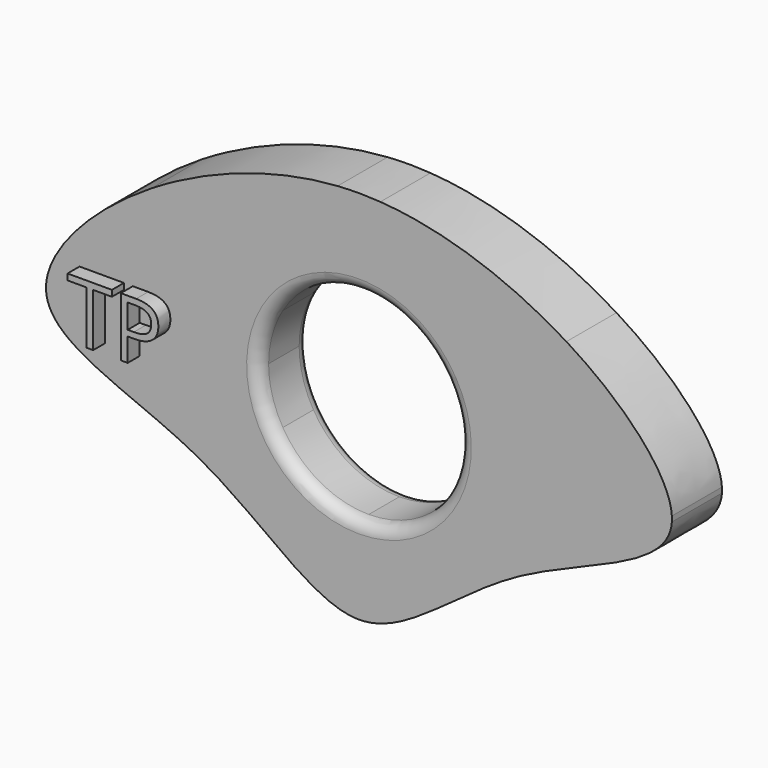
from build123d import *

# Parameters (mm, degrees)
F1_DEPTH     = 6.35
F3_TEXT_SIZE = 8.4123936378
F4_DEPTH     = 7.874


# Not quite as in the source:
# - a fillet or chamfer that OpenCascade refuses, or shapes differently, is made with other operations: its cross-section is extruded or revolved along the edge and cut away or added
# - Text() gives the source's letters only with a copy of the font that has no kerning and outlines rounded to 1/6400 em; it was checked with that copy


with BuildPart() as f1:
    # F0 (on Front) → F1 (new body)
    with BuildSketch(Plane.XZ):
        with BuildLine():
            add(Edge.make_bspline(
                [(-31.75, -38.1), (-26.9196709524, -38.1), (-22.0893419047, -32.5027306314), (-15.3722677145, -28.8766393713)],
                knots=[0.2929135327, 0.2929135327, 0.2929135327, 0.2929135327, 0.4404608065, 0.4404608065, 0.4404608065, 0.4404608065], degree=3))
            Line((-15.3722677145, -28.8766393713), (-23.0378718748, -24.2772768751))
            ThreePointArc((-23.0378718748, -24.2772768751), (-26.7441800398, -27.8912310526), (-31.75, -29.21))
            Line((-31.75, -29.21), (-31.75, -38.1))
        make_face()
        with BuildLine():
            ThreePointArc((-15.3722677145, -28.8766393713), (-13.3434748609, -24.148312314), (-12.6504461794, -19.05))
            Line((-12.6504461794, -19.05), (-21.59, -19.05))
            ThreePointArc((-21.59, -19.05), (-21.9586563294, -21.7620451921), (-23.0378718748, -24.2772768751))
            Line((-23.0378718748, -24.2772768751), (-15.3722677145, -28.8766393713))
        make_face()
        with BuildLine():
            add(Edge.make_bspline(
                [(-15.3722677145, -28.8766393713), (-8.7544839905, -25.3041482772), (-0.3053218561, -23.6449908652), (0, -19.05)],
                knots=[0.4404608065, 0.4404608065, 0.4404608065, 0.4404608065, 0.5858270655, 0.5858270655, 0.5858270655, 0.5858270655], degree=3))
            Line((0, -19.05), (-12.6504461794, -19.05))
            ThreePointArc((-12.6504461794, -19.05), (-13.3434748609, -24.148312314), (-15.3722677145, -28.8766393713))
        make_face()
        with BuildLine():
            Line((0, -19.05), (0, -18.5163144511))
            add(Edge.make_bspline(
                [(0, -18.5163144511), (-0.2161143448, -15.0824614861), (-4.4759800562, -10.2742950568), (-10.6970013922, -6.4182008353)],
                knots=[0.5913256791, 0.5913256791, 0.5913256791, 0.5913256791, 0.6951466037, 0.6951466037, 0.6951466037, 0.6951466037], degree=3))
            Line((-10.6970013922, -6.4182008353), (-15.3722677145, -9.2233606287))
            ThreePointArc((-15.3722677145, -9.2233606287), (-13.3434748609, -13.951687686), (-12.6504461794, -19.05))
            Line((-12.6504461794, -19.05), (0, -19.05))
        make_face()
        with BuildLine():
            ThreePointArc((-12.6504461794, -19.05), (-13.3434748609, -13.951687686), (-15.3722677145, -9.2233606287))
            Line((-15.3722677145, -9.2233606287), (-23.0378718748, -13.8227231249))
            ThreePointArc((-23.0378718748, -13.8227231249), (-21.9586563294, -16.3379548079), (-21.59, -19.05))
            Line((-21.59, -19.05), (-12.6504461794, -19.05))
        make_face()
        with BuildLine():
            add(Edge.make_bspline(
                [(-29.5779776849, -0.0743504667), (-30.3009796307, -0.025345087), (-31.0254898153, 0), (-31.75, 0)],
                knots=[0.783590155, 0.783590155, 0.783590155, 0.783590155, 0.7929135327, 0.7929135327, 0.7929135327, 0.7929135327], degree=3))
            Line((-31.75, 0), (-31.75, -8.89))
            ThreePointArc((-31.75, -8.89), (-26.7441800398, -10.2087689474), (-23.0378718748, -13.8227231249))
            Line((-23.0378718748, -13.8227231249), (-15.3722677145, -9.2233606287))
            ThreePointArc((-15.3722677145, -9.2233606287), (-21.4083634916, -2.9924936408), (-29.5779776849, -0.0743504667))
        make_face()
        with BuildLine():
            Line((-31.75, -8.89), (-31.75, 0))
            add(Edge.make_bspline(
                [(-31.75, 0), (-32.4745101847, 0), (-33.1990203693, -0.025345087), (-33.9220223151, -0.0743504667)],
                knots=[0.7929135327, 0.7929135327, 0.7929135327, 0.7929135327, 0.8022369105, 0.8022369105, 0.8022369105, 0.8022369105], degree=3))
            ThreePointArc((-33.9220223151, -0.0743504667), (-42.0916365084, -2.9924936408), (-48.1277322855, -9.2233606287))
            Line((-48.1277322855, -9.2233606287), (-40.4621281252, -13.8227231249))
            ThreePointArc((-40.4621281252, -13.8227231249), (-36.7558199602, -10.2087689474), (-31.75, -8.89))
        make_face()
        with BuildLine():
            ThreePointArc((-50.8495538206, -19.05), (-50.1565251391, -13.951687686), (-48.1277322855, -9.2233606287))
            Line((-48.1277322855, -9.2233606287), (-52.8029986078, -6.4182008353))
            add(Edge.make_bspline(
                [(-52.8029986078, -6.4182008353), (-59.0240199438, -10.2742950568), (-63.2838856552, -15.0824614861), (-63.5, -18.5163144511)],
                knots=[0.8906804618, 0.8906804618, 0.8906804618, 0.8906804618, 0.9945013864, 0.9945013864, 0.9945013864, 0.9945013864], degree=3))
            Line((-63.5, -18.5163144511), (-63.5, -19.05))
            Line((-63.5, -19.05), (-50.8495538206, -19.05))
        make_face()
        with BuildLine():
            ThreePointArc((-48.1277322855, -28.8766393713), (-50.1565251391, -24.148312314), (-50.8495538206, -19.05))
            Line((-50.8495538206, -19.05), (-63.5, -19.05))
            add(Edge.make_bspline(
                [(-63.5, -19.05), (-63.1946781439, -23.6449908652), (-54.7455160095, -25.3041482772), (-48.1277322855, -28.8766393713)],
                knots=[0, 0, 0, 0, 0.145366259, 0.145366259, 0.145366259, 0.145366259], degree=3))
        make_face()
        with BuildLine():
            Line((-48.1277322855, -28.8766393713), (-40.4621281252, -24.2772768751))
            ThreePointArc((-40.4621281252, -24.2772768751), (-41.5413436706, -21.7620451921), (-41.91, -19.05))
            Line((-41.91, -19.05), (-50.8495538206, -19.05))
            ThreePointArc((-50.8495538206, -19.05), (-50.1565251391, -24.148312314), (-48.1277322855, -28.8766393713))
        make_face()
        with BuildLine():
            ThreePointArc((-41.91, -19.05), (-41.5413436706, -16.3379548079), (-40.4621281252, -13.8227231249))
            Line((-40.4621281252, -13.8227231249), (-48.1277322855, -9.2233606287))
            ThreePointArc((-48.1277322855, -9.2233606287), (-50.1565251391, -13.951687686), (-50.8495538206, -19.05))
            Line((-50.8495538206, -19.05), (-41.91, -19.05))
        make_face()
        with BuildLine():
            add(Edge.make_bspline(
                [(-48.1277322855, -28.8766393713), (-41.4106580953, -32.5027306314), (-36.5803290476, -38.1), (-31.75, -38.1)],
                knots=[0.145366259, 0.145366259, 0.145366259, 0.145366259, 0.2929135327, 0.2929135327, 0.2929135327, 0.2929135327], degree=3))
            Line((-31.75, -38.1), (-31.75, -29.21))
            ThreePointArc((-31.75, -29.21), (-36.7558199602, -27.8912310526), (-40.4621281252, -24.2772768751))
            Line((-40.4621281252, -24.2772768751), (-48.1277322855, -28.8766393713))
        make_face()
        with BuildLine():
            Line((-15.3722677145, -9.2233606287), (-10.6970013922, -6.4182008353))
            add(Edge.make_bspline(
                [(-10.6970013922, -6.4182008353), (-15.9965999269, -3.1332496702), (-22.7194269191, -0.5392259577), (-29.5779776849, -0.0743504667)],
                knots=[0.6951466037, 0.6951466037, 0.6951466037, 0.6951466037, 0.783590155, 0.783590155, 0.783590155, 0.783590155], degree=3))
            ThreePointArc((-29.5779776849, -0.0743504667), (-21.4083634916, -2.9924936408), (-15.3722677145, -9.2233606287))
        make_face()
        with BuildLine():
            ThreePointArc((-48.1277322855, -9.2233606287), (-42.0916365084, -2.9924936408), (-33.9220223151, -0.0743504667))
            add(Edge.make_bspline(
                [(-33.9220223151, -0.0743504667), (-40.7805730809, -0.5392259577), (-47.5034000731, -3.1332496702), (-52.8029986078, -6.4182008353)],
                knots=[0.8022369105, 0.8022369105, 0.8022369105, 0.8022369105, 0.8906804618, 0.8906804618, 0.8906804618, 0.8906804618], degree=3))
            Line((-52.8029986078, -6.4182008353), (-48.1277322855, -9.2233606287))
        make_face()
    extrude(amount=F1_DEPTH)

    # F2: fillet of radius 1.27 on 2 edges, made by hand

    # F2_s1 → F2_t2 (revolve, cut)
    with BuildSketch(Plane.YZ.offset(-31.75)):
        with BuildLine():
            ThreePointArc((-5.0790343146, -29.2096), (-5.9780256121, -29.5819743879), (-6.3504, -30.4809656854))
            Line((-6.3504, -30.4809656854), (-6.4775365685, -30.4809656854))
            ThreePointArc((-6.4775365685, -30.4809656854), (-6.4771365685, -29.8454828427), (-6.4771365685, -29.21))
            Line((-6.4771365685, -29.21), (-6.35, -29.0828634315))
            ThreePointArc((-6.35, -29.0828634315), (-5.7145171573, -29.0828634315), (-5.0790343146, -29.0824634315))
            Line((-5.0790343146, -29.0824634315), (-5.0790343146, -29.2096))
        make_face()
    revolve(axis=Axis((-31.75, -6.35, -19.05), (0, 1, 0)), mode=Mode.SUBTRACT)

    # F2_s3 → F2_t4 (revolve, cut)
    with BuildSketch(Plane.YZ.offset(-31.75)):
        with BuildLine():
            ThreePointArc((-1.2709656854, -29.2096), (-0.3719743879, -29.5819743879), (0.0004, -30.4809656854))
            Line((0.0004, -30.4809656854), (0.1275365685, -30.4809656854))
            ThreePointArc((0.1275365685, -30.4809656854), (0.1271365685, -29.8454828427), (0.1271365685, -29.21))
            Line((0.1271365685, -29.21), (0, -29.0828634315))
            ThreePointArc((0, -29.0828634315), (-0.6354828427, -29.0828634315), (-1.2709656854, -29.0824634315))
            Line((-1.2709656854, -29.0824634315), (-1.2709656854, -29.2096))
        make_face()
    revolve(axis=Axis((-31.75, 0, -19.05), (0, 1, 0)), mode=Mode.SUBTRACT)

    # F3 (on Front) → F4 (join)
    with BuildSketch(Plane.XZ):
        with Locations((-60.1784624159, -21.7853859067)):
            Text('TP', F3_TEXT_SIZE, font='Open Sans', text_align=(TextAlign.LEFT, TextAlign.BOTTOM))
    extrude(amount=F4_DEPTH)


solid = f1.part
